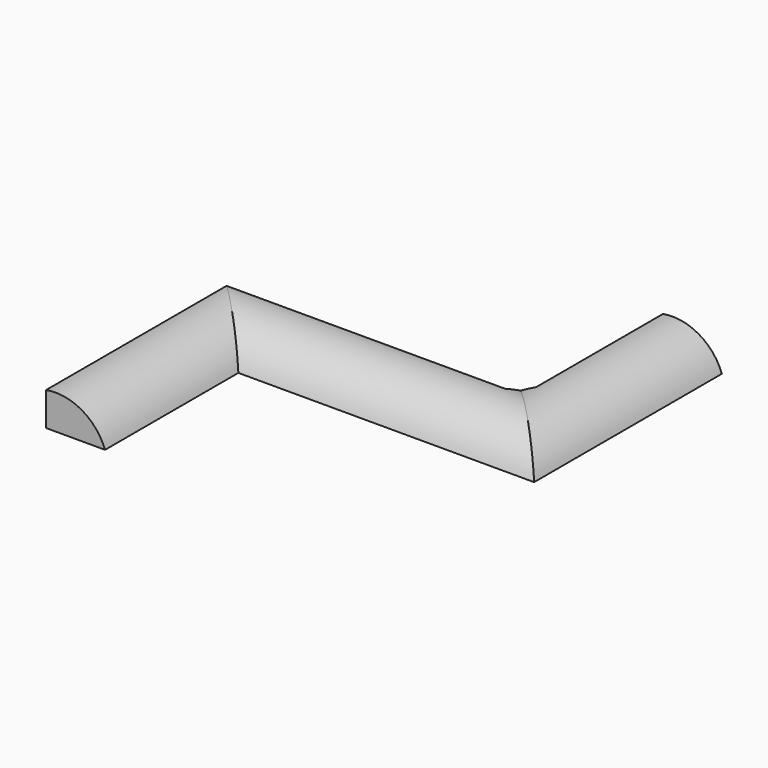
from build123d import *

# Parameters (mm, degrees)
F3_T4_DEPTH  = 67.761612304
F3_S5_R      = 45.861643493
F3_T6_DEPTH  = 37
F3_S7_R      = 45.861643493
F3_T8_DEPTH  = 37
F3_T12_DEPTH = 67.761612304
F3_S13_R     = 45.861643493
F3_T14_DEPTH = 37
F3_S15_R     = 45.861643493
F3_T16_DEPTH = 37
F3_T20_DEPTH = 67.761612304
F3_S21_R     = 45.861643493
F3_T22_DEPTH = 37
F3_S23_R     = 45.861643493
F3_T24_DEPTH = 37


# Not quite as in the source:
# - a fillet or chamfer that OpenCascade refuses, or shapes differently, is made with other operations: its cross-section is extruded or revolved along the edge and cut away or added


with BuildPart() as f2:
    # F2: sweep along a path in F1
    with BuildLine(Plane.XY) as f2_path:
        Line((0, 0), (0, -153.106674552))
        Line((0, -153.106674552), (-257.6704025269, -153.106674552))
        Line((-257.6704025269, -153.106674552), (-257.6704025269, -349.6235013008))
    # F0 (on Front) → F2 (sweep)
    with BuildSketch(Plane.XZ):
        with BuildLine():
            Line((0, 0), (44.372734969, 0))
            add(Edge.make_bspline(
                [(44.372734969, 0), (44.372734969, 22.1863674845), (0, 22.1863674845)],
                knots=[3.1415926536, 3.1415926536, 3.1415926536, 4.7123889804, 4.7123889804, 4.7123889804], degree=2, weights=[1, 0.7071067812, 1]))
            Line((0, 22.1863674845), (0, 0))
        make_face()
        with BuildLine():
            add(Edge.make_bspline(
                [(44.372734969, 0), (44.372734969, 22.1863674845), (0, 22.1863674845)],
                knots=[3.1415926536, 3.1415926536, 3.1415926536, 4.7123889804, 4.7123889804, 4.7123889804], degree=2, weights=[1, 0.7071067812, 1]))
            Line((44.372734969, 0), (51.372734969, 0))
            ThreePointArc((51.372734969, 0), (31.0126987208, 23.9683895846), (0, 29.1863674845))
            Line((0, 29.1863674845), (0, 22.1863674845))
        make_face()
    sweep(path=f2_path.line, transition=Transition.RIGHT)

    # F3: chamfer of 15 on 1 edges, made by hand


with BuildPart() as f3_tool2:
    # F3_s3 → F3_t4 (new body)
    with BuildSketch(Plane.XY):
        Polygon((0, -138.106674552), (-15, -153.106674552), (0, -153.106674552), align=None)
    extrude(amount=F3_T4_DEPTH)

    # F3_s5 → F3_t6 (intersect, symmetric)
    with BuildSketch(Plane.XZ.offset(145.6)):
        with Locations((8.3581917564, -15.9072127065)):
            Circle(F3_S5_R)
    extrude(amount=F3_T6_DEPTH, both=True, mode=Mode.INTERSECT)

    # F3_s7 → F3_t8 (intersect, symmetric)
    with BuildSketch(Plane.YZ.offset(-7.5)):
        with Locations((-161.4648663084, -15.9072127065)):
            Circle(F3_S7_R)
    extrude(amount=F3_T8_DEPTH, both=True, mode=Mode.INTERSECT)


with BuildPart() as f2_1:
    add(f2.part)

    # F3_t1: union F3_tool2
    add(f3_tool2.part)


with BuildPart() as f3_tool10:
    # F3_s11 → F3_t12 (new body)
    with BuildSketch(Plane.XY):
        Polygon((0, -138.106674552), (-15, -153.106674552), (0, -153.106674552), align=None)
    extrude(amount=F3_T12_DEPTH)

    # F3_s13 → F3_t14 (cut, symmetric)
    with BuildSketch(Plane.XZ.offset(145.6)):
        with Locations((8.3581917564, -15.9072127065)):
            Circle(F3_S13_R)
    extrude(amount=F3_T14_DEPTH, both=True, mode=Mode.SUBTRACT)

    # F3_s15 → F3_t16 (intersect, symmetric)
    with BuildSketch(Plane.YZ.offset(-7.5)):
        with Locations((-161.4648663084, -15.9072127065)):
            Circle(F3_S15_R)
    extrude(amount=F3_T16_DEPTH, both=True, mode=Mode.INTERSECT)


with BuildPart() as f2_2:
    add(f2_1.part)

    # F3_t9: union F3_tool10
    add(f3_tool10.part)


with BuildPart() as f3_tool18:
    # F3_s19 → F3_t20 (new body)
    with BuildSketch(Plane.XY):
        Polygon((0, -138.106674552), (-15, -153.106674552), (0, -153.106674552), align=None)
    extrude(amount=F3_T20_DEPTH)

    # F3_s21 → F3_t22 (intersect, symmetric)
    with BuildSketch(Plane.XZ.offset(145.6)):
        with Locations((8.3581917564, -15.9072127065)):
            Circle(F3_S21_R)
    extrude(amount=F3_T22_DEPTH, both=True, mode=Mode.INTERSECT)

    # F3_s23 → F3_t24 (cut, symmetric)
    with BuildSketch(Plane.YZ.offset(-7.5)):
        with Locations((-161.4648663084, -15.9072127065)):
            Circle(F3_S23_R)
    extrude(amount=F3_T24_DEPTH, both=True, mode=Mode.SUBTRACT)


with BuildPart() as f2_3:
    add(f2_2.part)

    # F3_t17: union F3_tool18
    add(f3_tool18.part)


solid = f2_3.part
